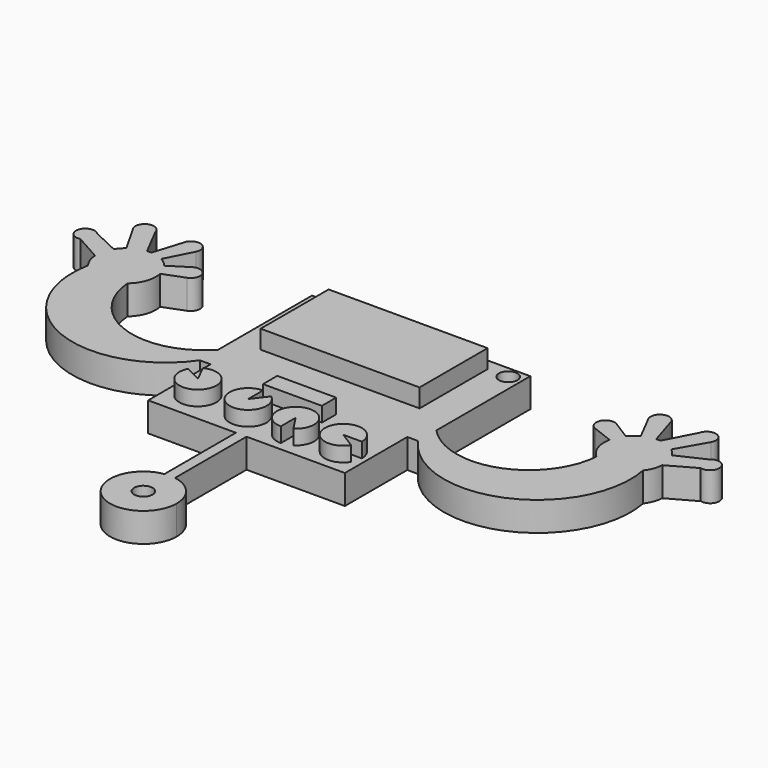
from build123d import *

# Parameters (mm, degrees)
F0_R     = 4.2534442679
F1_DEPTH = 20
F2_W     = 10.3906942531
F2_H     = 12.2660957277
F2_W_2   = 9.8304990679
F2_W_3   = 9.2522380874
F2_W_4   = 10.9689552337
F3_DEPTH = 10.16
F5_R     = 6.35
F6_DEPTH = 25.4
F7_R     = 6.35
F8_DEPTH = 25.4
F4_W     = 109.22
F4_H     = 58.420000254
F9_DEPTH = 12.7


# Not quite as in the source:
# - a feature names something its author has since deleted; it is built from what else it names


with BuildPart() as f1:
    # F0 (on Top) → F1 (new body)
    with BuildSketch(Plane.XY):
        Polygon((-67.5837442279, -21.374759078), (-67.5837442279, -75), (-7.2734476998, -75), (0, -75), (67.5837334, -75), (67.5837334, -21.374759078), (75, -21.374759078), (75, -5.6661395316), (75, 75), (-75, 75), (-75, -5.6661395316), (-75, -21.374759078), align=None)
        with BuildLine():
            ThreePointArc((-190.7009859405, 27.2364963511), (-152.5558792144, -43.9704630954), (-75, -21.374759078))
            Line((-75, -21.374759078), (-75, -5.6661395316))
            ThreePointArc((-75, -5.6661395316), (-127.811049195, -18.8460311242), (-161.148882109, 24.1807669913))
            ThreePointArc((-161.148882109, 24.1807669913), (-155.1100282823, 33.0940415029), (-154.4303864618, 43.8389149342))
            Line((-154.4303864618, 43.8389149342), (-140.2046696458, 49.3057770206))
            ThreePointArc((-140.2046696458, 49.3057770206), (-136.7560169722, 57.9771637157), (-145.6751462177, 60.7222112528))
            Line((-145.6751462177, 60.7222112528), (-146.0841166448, 60.4629836272))
            Line((-146.0841166448, 60.4629836272), (-158.5471573729, 52.5632328352))
            ThreePointArc((-158.5471573729, 52.5632328352), (-161.385975302, 55.4455313061), (-164.7362764103, 57.7131322838))
            Line((-164.7362764103, 57.7131322838), (-155.482622785, 75.8038009996))
            ThreePointArc((-155.482622785, 75.8038009996), (-159.2281719938, 84.7522052149), (-167.4260348338, 79.5658652979))
            Line((-167.4260348338, 79.5658652979), (-173.4289959882, 60.1528063587))
            ThreePointArc((-173.4289959882, 60.1528063587), (-174.9118696964, 60.1750253912), (-176.3924593558, 60.0898057902))
            Line((-176.3924593558, 60.0898057902), (-186.9047044679, 80.3893698915))
            ThreePointArc((-186.9047044679, 80.3893698915), (-195.4793934942, 84.7270210192), (-198.5276463049, 75.6139170472))
            Line((-198.5276463049, 75.6139170472), (-187.1383609375, 55.7931254681))
            ThreePointArc((-187.1383609375, 55.7931254681), (-189.6692112484, 53.4271036789), (-191.7647204388, 50.6680995766))
            Line((-191.7647204388, 50.6680995766), (-210.142074272, 59.3384667019))
            ThreePointArc((-210.142074272, 59.3384667019), (-220.775202398, 56.5846111171), (-213.1234756292, 48.7043692565))
            Line((-213.1234756292, 48.7043692565), (-194.9065059539, 38.4823538939))
            ThreePointArc((-194.9065059539, 38.4823538939), (-193.6469430671, 32.5441016935), (-190.7009859405, 27.2364963511))
        make_face()
        with BuildLine():
            Line((75, -5.6661395316), (75, -21.374759078))
            ThreePointArc((75, -21.374759078), (152.5558792144, -43.9704630954), (190.7009859405, 27.2364963511))
            ThreePointArc((190.7009859405, 27.2364963511), (193.6469430671, 32.5441016935), (194.9065059539, 38.4823538939))
            Line((194.9065059539, 38.4823538939), (213.1234756292, 48.7043692565))
            ThreePointArc((213.1234756292, 48.7043692565), (220.775202398, 56.5846111171), (210.142074272, 59.3384667019))
            Line((210.142074272, 59.3384667019), (191.7647204388, 50.6680995766))
            ThreePointArc((191.7647204388, 50.6680995766), (189.6692112484, 53.4271036789), (187.1383609375, 55.7931254681))
            Line((187.1383609375, 55.7931254681), (198.5276463049, 75.6139170472))
            ThreePointArc((198.5276463049, 75.6139170472), (195.4793934942, 84.7270210192), (186.9047044679, 80.3893698915))
            Line((186.9047044679, 80.3893698915), (176.3924593558, 60.0898057902))
            ThreePointArc((176.3924593558, 60.0898057902), (174.9118696964, 60.1750253912), (173.4289959882, 60.1528063587))
            Line((173.4289959882, 60.1528063587), (167.4260348338, 79.5658652979))
            ThreePointArc((167.4260348338, 79.5658652979), (159.2281719938, 84.7522052149), (155.482622785, 75.8038009996))
            Line((155.482622785, 75.8038009996), (164.7362764103, 57.7131322838))
            ThreePointArc((164.7362764103, 57.7131322838), (161.385975302, 55.4455313061), (158.5471573729, 52.5632328352))
            Line((158.5471573729, 52.5632328352), (146.0841166448, 60.4629836272))
            Line((146.0841166448, 60.4629836272), (145.6751462177, 60.7222112528))
            ThreePointArc((145.6751462177, 60.7222112528), (136.7560169722, 57.9771637157), (140.2046696458, 49.3057770206))
            Line((140.2046696458, 49.3057770206), (154.4303864618, 43.8389149342))
            ThreePointArc((154.4303864618, 43.8389149342), (155.1100282823, 33.0940415029), (161.148882109, 24.1807669913))
            ThreePointArc((161.148882109, 24.1807669913), (127.811049195, -18.8460311242), (75, -5.6661395316))
        make_face()
        with BuildLine():
            Line((0, -75), (-7.2734476998, -75))
            Line((-7.2734476998, -75), (-7.2734476998, -136.4104553148))
            ThreePointArc((-7.2734476998, -136.4104553148), (-3.6367238499, -136.120270713), (0, -136.4104553148))
            Line((0, -136.4104553148), (0, -75))
        make_face()
        with BuildLine():
            ThreePointArc((0, -136.4104553148), (-3.6367238499, -136.120270713), (-7.2734476998, -136.4104553148))
            ThreePointArc((-7.2734476998, -136.4104553148), (-18.5120008809, -176.508894443), (19.2968973343, -159.0538918972))
            ThreePointArc((19.2968973343, -159.0538918972), (13.8182786959, -144.1786148662), (0, -136.4104553148))
        make_face()
        with Locations((-3.6367238499, -159.0538918972)):
            Circle(F0_R, mode=Mode.SUBTRACT)
        with Locations((-3.6367238499, -159.0538918972)):
            Circle(F0_R)
    extrude(amount=F1_DEPTH)

    # F2 (on face) → F3 (join)
    with BuildSketch(Plane.XY.offset(20)):
        with Locations((-13.8693177141, -30.8799799532)):
            Rectangle(F2_W, F2_H)
        with Locations((-3.7587210536, -30.8799799532)):
            Rectangle(F2_W_2, F2_H)
        with Locations((5.782647524, -30.8799799532)):
            Rectangle(F2_W_3, F2_H)
        with Locations((15.8932441846, -30.8799799532)):
            Rectangle(F2_W_4, F2_H)
        with BuildLine():
            Line((-50.2273030579, -53.9529807866), (-61.5431257083, -48.187379539))
            ThreePointArc((-61.5431257083, -48.187379539), (-41.2897769448, -62.9757645575), (-55.8852143831, -42.5829306795))
            Line((-55.8852143831, -42.5829306795), (-50.2273030579, -53.9529807866))
        make_face()
        with BuildLine():
            Line((-14.4444061443, -55.5018670857), (-14.4444061443, -42.8018670857))
            ThreePointArc((-14.4444061443, -42.8018670857), (-18.5320544995, -67.5260564939), (-6.7041450331, -45.4331850503))
            Line((-6.7041450331, -45.4331850503), (-14.4444061443, -55.5018670857))
        make_face()
        with BuildLine():
            Line((19.0666168928, -56.657422334), (26.0705094181, -67.2515475689))
            ThreePointArc((26.0705094181, -67.2515475689), (15.4098006877, -44.4952804485), (19.0666168928, -69.357422334))
            Line((19.0666168928, -69.357422334), (19.0666168928, -56.657422334))
        make_face()
        with BuildLine():
            Line((51.4220893383, -56.0796447098), (64.1220893383, -56.0796447098))
            ThreePointArc((64.1220893383, -56.0796447098), (39.2223619287, -52.550246584), (62.1604119949, -62.8603840886))
            Line((62.1604119949, -62.8603840886), (51.4220893383, -56.0796447098))
        make_face()
    extrude(amount=F3_DEPTH)

    # F5 (on face) → F6 (cut)
    with BuildSketch(Plane.XY.offset(20)):
        with Locations((-3.6367238499, -159.0538918972)):
            Circle(F5_R)
    extrude(amount=-F6_DEPTH, mode=Mode.SUBTRACT)

    # F7 (on face) → F8 (cut)
    with BuildSketch(Plane.XY.offset(20)):
        with Locations((66.185079515, 67.0784339309)):
            Circle(F7_R)
    extrude(amount=-F8_DEPTH, mode=Mode.SUBTRACT)

    # F4 (on face) → F9 (join)
    with BuildSketch(Plane.XY.offset(20)):
        with Locations((-2.614335165, 37.8684338039)):
            Rectangle(F4_W, F4_H)
    extrude(amount=F9_DEPTH)


solid = f1.part
